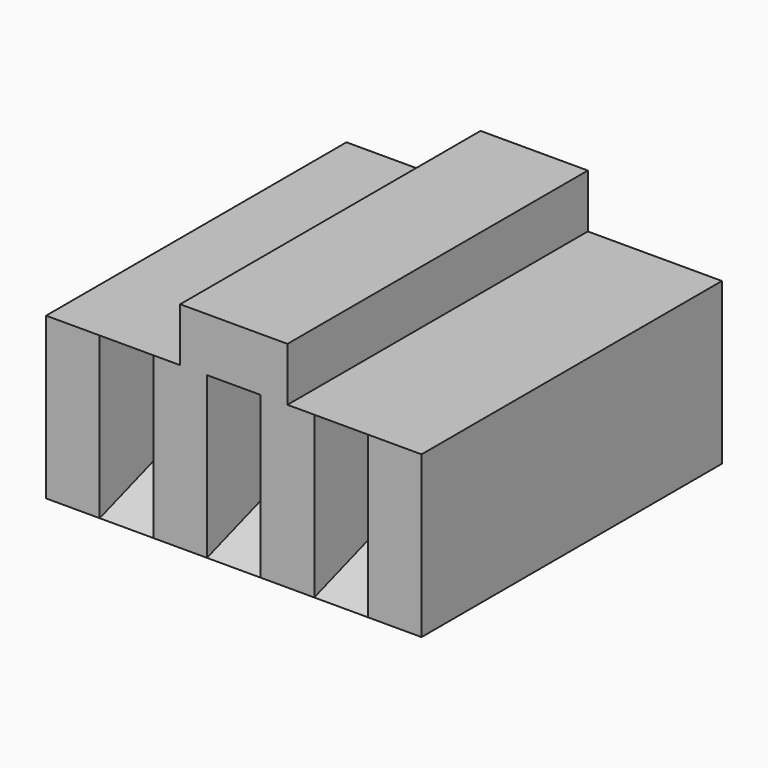
from build123d import *

# Parameters (mm, degrees)
F0_W       = 1
F0_H       = 1
F1_DEPTH   = 7
F2_SIZE2   = 2.747467
F2_SIZE    = 0.99999
F2_2_SIZE2 = 2.747467
F2_2_SIZE  = 0.99999
F3_SIZE2   = 2.904201
F3_SIZE    = 0.99999


# Not quite as in the source:
# - a fillet or chamfer is up to 0.001 mm smaller than in the source, because OpenCascade refuses the exact size


with BuildPart() as f1:
    # F0 (on Front) → F1 (new body)
    with BuildSketch(Plane.XZ):
        Polygon((-56.745035848, 28.2884484402), (-56.745035848, 26.7884484402), (-56.745035848, 25.2884484402), (-51.245035848, 25.2884484402), (-51.245035848, 26.2884484402), (-51.745035848, 26.2884484402), (-51.745035848, 27.2884484402), (-51.245035848, 27.2884484402), (-51.245035848, 28.2884484402), (-52.245035848, 28.2884484402), (-53.245035848, 28.2884484402), (-54.245035848, 28.2884484402), align=None)
        Polygon((-54.745035848, 26.2884484402), (-55.745035848, 26.2884484402), (-55.745035848, 26.7884484402), (-55.745035848, 27.2884484402), (-54.745035848, 27.2884484402), align=None, mode=Mode.SUBTRACT)
        with Locations((-53.245035848, 26.7884484402)):
            Rectangle(F0_W, F0_H, mode=Mode.SUBTRACT)
        Polygon((-50.745035848, 26.7884484402), (-49.745035848, 26.7884484402), (-49.745035848, 28.2884484402), (-51.245035848, 28.2884484402), (-51.245035848, 27.2884484402), (-50.745035848, 27.2884484402), align=None)
        Polygon((-51.245035848, 26.2884484402), (-51.245035848, 25.2884484402), (-49.745035848, 25.2884484402), (-49.745035848, 26.7884484402), (-50.745035848, 26.7884484402), (-50.745035848, 26.2884484402), align=None)
        with Locations((-52.745035848, 28.7884484402)):
            Rectangle(F0_W, F0_H)
        with Locations((-53.745035848, 28.7884484402)):
            Rectangle(F0_W, F0_H)
    extrude(amount=F1_DEPTH)

    # F2 (size 1 and 2.7474774195 in the source; OpenCascade refuses exactly that, so slightly less here)
    f2_edges = [f1.edges().sort_by_distance(p)[0] for p in [
        (-51.245036, 0, 26.288448),
        (-51.245036, 0, 27.288448),
        (-53.245036, 0, 27.288448),
        (-53.245036, 0, 26.288448),
        (-55.245036, 0, 27.288448),
        (-55.245036, 0, 26.288448),
    ]]
    f2_side = f1.faces().sort_by_distance((-56.664413, 0, 26.788448))[0]
    chamfer(f2_edges, length=F2_SIZE, length2=F2_SIZE2, reference=f2_side)

    # F2#2 (size 1 and 2.7474774195 in the source; OpenCascade refuses exactly that, so slightly less here)
    f2_2_edges = [f1.edges().sort_by_distance(p)[0] for p in [
        (-55.245036, -7, 27.288448),
        (-53.245036, -7, 27.288448),
        (-51.245036, -7, 27.288448),
    ]]
    f2_2_side = f1.faces().sort_by_distance((-56.664413, -7, 26.788448))[0]
    chamfer(f2_2_edges, length=F2_2_SIZE, length2=F2_2_SIZE2, reference=f2_2_side)

    # F3 (size 1 and 2.9042108777 in the source; OpenCascade refuses exactly that, so slightly less here)
    f3_edges = [f1.edges().sort_by_distance(p)[0] for p in [
        (-55.245036, -7, 26.288448),
        (-53.245036, -7, 26.288448),
        (-51.245036, -7, 26.288448),
    ]]
    f3_side = f1.faces().sort_by_distance((-55.825658, -7, 27.788443))[0]
    chamfer(f3_edges, length=F3_SIZE, length2=F3_SIZE2, reference=f3_side)


solid = f1.part
